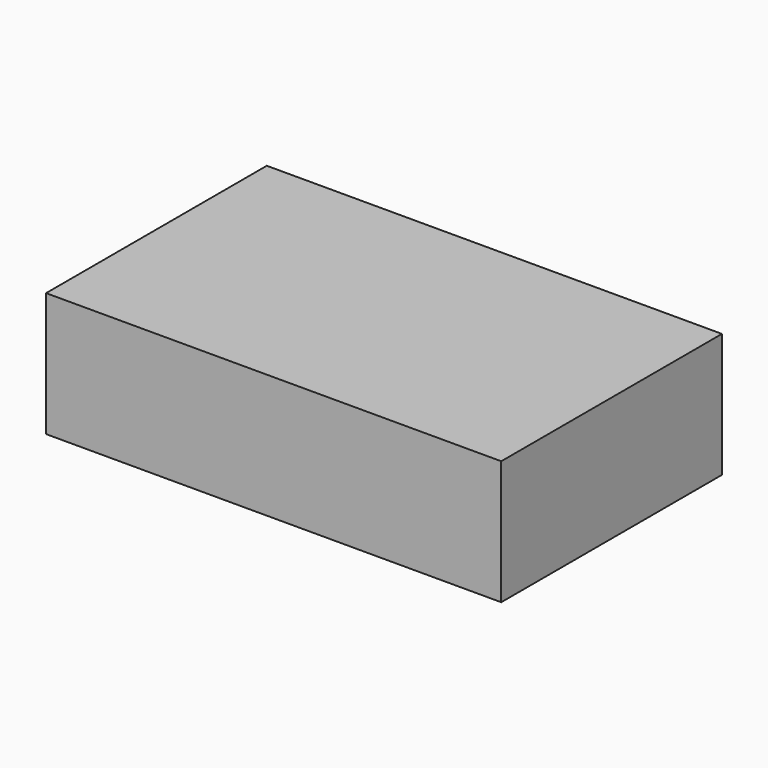
from build123d import *

# Parameters (mm, degrees)
F0_W     = 330
F0_H     = 60
F0_H_2   = 34.9986995305
F0_H_3   = 105.0013004695
F1_DEPTH = 90


with BuildPart() as f1:
    # F0 (on Top) → F1 (new body)
    with BuildSketch(Plane.XY):
        with Locations((-1.3739347196, -104.1871940094)):
            Rectangle(F0_W, F0_H)
        with Locations((-1.3739347196, -56.6878442441)):
            Rectangle(F0_W, F0_H_2)
        with Locations((-1.3739347196, 13.3121557559)):
            Rectangle(F0_W, F0_H_3)
    extrude(amount=F1_DEPTH)


solid = f1.part
